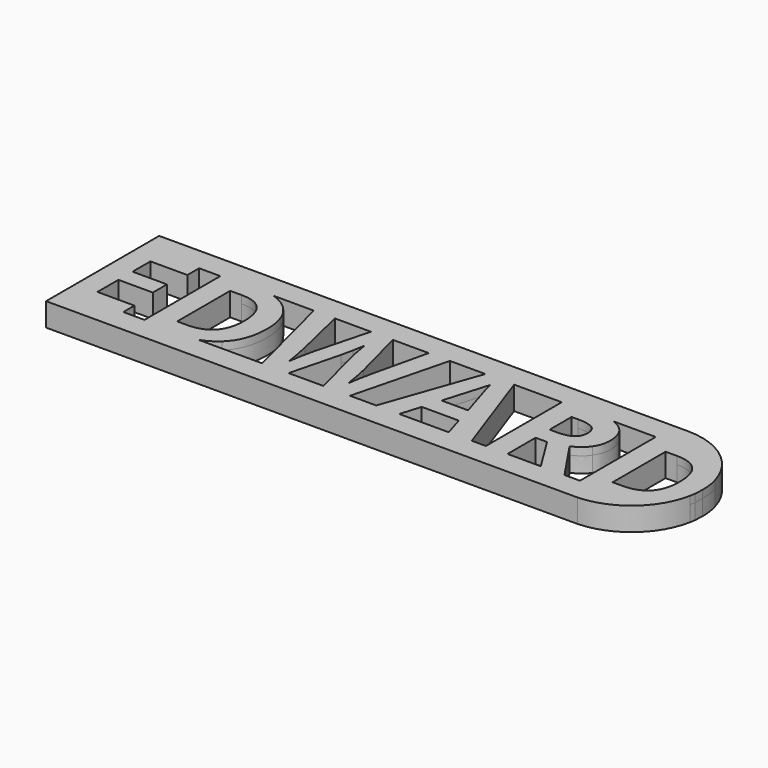
from build123d import *

# Parameters (mm, degrees)
F0_W     = 7.5354432192
F0_H     = 0.5
F0_W_2   = 2.7753114707
F0_H_2   = 0.3883001575
F1_DEPTH = 2
F2_DEPTH = 1.6468566519
F3_DEPTH = 1.6468566519
F5_DEPTH = 2
F6_DEPTH = 2
F7_DEPTH = 1


with BuildPart() as f1:
    # F0 (on Top) → F1 (new body)
    with BuildSketch(Plane.XY):
        with Locations((-34.5854217385, 0.25)):
            Rectangle(F0_W, F0_H)
        Polygon((-38.3531433481, 12.6977660032), (-38.3531433481, 0.5), (-30.8177001289, 0.5), (-30.8177001289, 2.29127882), (-35.5778318774, 2.29127882), (-35.5778318774, 5.6651868824), (-31.1470714593, 5.6651868824), (-31.1470714593, 7.9392811113), (-35.5778318774, 7.9392811113), (-35.5778318774, 10.8119719318), (-30.8177001289, 10.8119719318), (-30.8177001289, 12.6977660032), align=None)
        with BuildLine():
            Line((-38.3531433481, 0.5), (-40, 0.5))
            Line((-40, 0.5), (-40, -2.5))
            Line((-40, -2.5), (40, -2.5))
            Line((40, -2.5), (40, 0.5))
            Line((40, 0.5), (34.9300250632, 0.5))
            add(Edge.make_bspline(
                [(34.9300250632, 0.5), (33.5321767459, 0), (31.6597450952, 0)],
                knots=[0.460594463, 0.460594463, 0.460594463, 1, 1, 1], degree=2))
            Line((31.6597450952, 0), (27.9536016039, 0))
            Line((27.9536016039, 0), (27.9536016039, 0.5))
            Line((27.9536016039, 0.5), (25.9628201622, 0.5))
            add(Edge.make_bspline(
                [(25.9628201622, 0.5), (26.1618801681, 0.2089395921), (26.306744952, 0)],
                knots=[0.837886092, 0.837886092, 0.837886092, 1, 1, 1], degree=2))
            Line((26.306744952, 0), (23.2278390377, 0))
            Line((23.2278390377, 0), (22.9166582048, 0.5))
            Line((22.9166582048, 0.5), (18.6280968065, 0.5))
            Line((18.6280968065, 0.5), (18.6280968065, 0))
            Line((18.6280968065, 0), (15.8527853358, 0))
            Line((15.8527853358, 0), (15.8527853358, 0.5))
            Line((15.8527853358, 0.5), (14.0294901486, 0.5))
            Line((14.0294901486, 0.5), (14.2059286839, 0))
            Line((14.2059286839, 0), (11.2158098239, 0))
            Line((11.2158098239, 0), (11.0636958533, 0.5))
            Line((11.0636958533, 0.5), (4.7003024283, 0.5))
            Line((4.7003024283, 0.5), (4.5481884577, 0))
            Line((4.5481884577, 0), (1.5580695976, 0))
            Line((1.5580695976, 0), (1.7338542532, 0.5))
            Line((1.7338542532, 0.5), (-1.6456062494, 0.5))
            Line((-1.6456062494, 0.5), (-1.772876987, 0))
            Line((-1.772876987, 0), (-4.93197766, 0))
            Line((-4.93197766, 0), (-5.0609359934, 0.5))
            Line((-5.0609359934, 0.5), (-9.5464787021, 0.5))
            Line((-9.5464787021, 0.5), (-9.6749248174, 0))
            Line((-9.6749248174, 0), (-12.8254331949, 0))
            Line((-12.8254331949, 0), (-12.9530322319, 0.5))
            Line((-12.9530322319, 0.5), (-21.1117907752, 0.5))
            add(Edge.make_bspline(
                [(-21.1117907752, 0.5), (-22.5096390926, 0), (-24.3820707432, 0)],
                knots=[0.460594463, 0.460594463, 0.460594463, 1, 1, 1], degree=2))
            Line((-24.3820707432, 0), (-28.0882142346, 0))
            Line((-28.0882142346, 0), (-28.0882142346, 0.5))
            Line((-28.0882142346, 0.5), (-30.8177001289, 0.5))
            Line((-30.8177001289, 0.5), (-30.8177001289, 0))
            Line((-30.8177001289, 0), (-38.3531433481, 0))
            Line((-38.3531433481, 0), (-38.3531433481, 0.5))
        make_face()
        with BuildLine():
            Line((-28.0882142346, 12.6977660032), (-28.0882142346, 0.5))
            Line((-28.0882142346, 0.5), (-21.1117907752, 0.5))
            add(Edge.make_bspline(
                [(-19.0706000286, 1.718459115), (-19.9181782686, 0.9269463617), (-21.1117907752, 0.5)],
                knots=[0, 0, 0, 0.460594463, 0.460594463, 0.460594463], degree=2))
            add(Edge.make_bspline(
                [(-17.2304167263, 6.6676213662), (-17.2304167263, 3.43691823), (-19.0706000286, 1.718459115)],
                knots=[0, 0, 0, 1, 1, 1], degree=2))
            add(Edge.make_bspline(
                [(-19.0032937133, 11.3948159817), (-17.2304167263, 9.7035658027), (-17.2304167263, 6.6676213662)],
                knots=[0, 0, 0, 1, 1, 1], degree=2))
            add(Edge.make_bspline(
                [(-21.2385462766, 12.6977660032), (-19.9266803337, 12.2756880323), (-19.0032937133, 11.3948159817)],
                knots=[0.479159227, 0.479159227, 0.479159227, 1, 1, 1], degree=2))
            Line((-21.2385462766, 12.6977660032), (-28.0882142346, 12.6977660032))
        make_face()
        with BuildLine():
            add(Edge.make_bspline(
                [(-20.114563941, 6.5960189031), (-20.114563941, 10.8119719318), (-23.8378920235, 10.8119719318)],
                knots=[0, 0, 0, 1, 1, 1], degree=2))
            add(Edge.make_bspline(
                [(-24.124301876, 2.29127882), (-20.114563941, 2.29127882), (-20.114563941, 6.5960189031)],
                knots=[0, 0, 0, 1, 1, 1], degree=2))
            Line((-24.124301876, 2.29127882), (-25.3129027639, 2.29127882))
            Line((-25.3129027639, 2.29127882), (-25.3129027639, 10.8119719318))
            Line((-25.3129027639, 10.8119719318), (-23.8378920235, 10.8119719318))
        make_face(mode=Mode.SUBTRACT)
        with BuildLine():
            Line((-21.1117907752, 0.5), (-28.0882142346, 0.5))
            Line((-28.0882142346, 0.5), (-28.0882142346, 0))
            Line((-28.0882142346, 0), (-24.3820707432, 0))
            add(Edge.make_bspline(
                [(-21.1117907752, 0.5), (-22.5096390926, 0), (-24.3820707432, 0)],
                knots=[0.460594463, 0.460594463, 0.460594463, 1, 1, 1], degree=2))
        make_face()
        with BuildLine():
            Line((-16.0658786227, 12.6977660032), (-12.9530322319, 0.5))
            Line((-12.9530322319, 0.5), (-9.5464787021, 0.5))
            Line((-9.5464787021, 0.5), (-7.9135042245, 6.8566518688))
            add(Edge.make_bspline(
                [(-7.5812687956, 8.3817843334), (-7.796076185, 7.3120435343), (-7.9135042245, 6.8566518688)],
                knots=[0, 0, 0, 1, 1, 1], degree=2))
            add(Edge.make_bspline(
                [(-7.3120435343, 9.9355577832), (-7.3664614063, 9.4515251325), (-7.5812687956, 8.3817843334)],
                knots=[0, 0, 0, 1, 1, 1], degree=2))
            add(Edge.make_bspline(
                [(-7.0399541744, 8.390376629), (-7.277674352, 9.5403121867), (-7.3120435343, 9.9355577832)],
                knots=[0, 0, 0, 1, 1, 1], degree=2))
            add(Edge.make_bspline(
                [(-6.704854647, 6.87383646), (-6.8022339968, 7.2404410712), (-7.0399541744, 8.390376629)],
                knots=[0, 0, 0, 1, 1, 1], degree=2))
            Line((-6.704854647, 6.87383646), (-5.0609359934, 0.5))
            Line((-5.0609359934, 0.5), (-1.6456062494, 0.5))
            Line((-1.6456062494, 0.5), (1.4592311027, 12.6977660032))
            Line((1.4592311027, 12.6977660032), (-1.2647384512, 12.6977660032))
            Line((-1.2647384512, 12.6977660032), (-2.8383216383, 5.9430044394))
            add(Edge.make_bspline(
                [(-3.1963339539, 4.2560504081), (-2.9987111557, 5.2985822712), (-2.8383216383, 5.9430044394)],
                knots=[0, 0, 0, 1, 1, 1], degree=2))
            add(Edge.make_bspline(
                [(-3.4827438064, 2.5146785049), (-3.3939567521, 3.213518545), (-3.1963339539, 4.2560504081)],
                knots=[0, 0, 0, 1, 1, 1], degree=2))
            add(Edge.make_bspline(
                [(-3.7677216096, 4.2517542603), (-3.5801231562, 3.2392954318), (-3.4827438064, 2.5146785049)],
                knots=[0, 0, 0, 1, 1, 1], degree=2))
            add(Edge.make_bspline(
                [(-4.0813403981, 5.7539739367), (-3.955320063, 5.2642130889), (-3.7677216096, 4.2517542603)],
                knots=[0, 0, 0, 1, 1, 1], degree=2))
            Line((-4.0813403981, 5.7539739367), (-5.8878113029, 12.6977660032))
            Line((-5.8878113029, 12.6977660032), (-8.710498879, 12.6977660032))
            Line((-8.710498879, 12.6977660032), (-10.5169697838, 5.7539739367))
            add(Edge.make_bspline(
                [(-10.8792782472, 4.0942288415), (-10.6859515967, 5.1639696406), (-10.5169697838, 5.7539739367)],
                knots=[0, 0, 0, 1, 1, 1], degree=2))
            add(Edge.make_bspline(
                [(-11.1270227696, 2.5146785049), (-11.0726048976, 3.0244880424), (-10.8792782472, 4.0942288415)],
                knots=[0, 0, 0, 1, 1, 1], degree=2))
            add(Edge.make_bspline(
                [(-11.7599885436, 5.9430044394), (-11.3217814693, 3.9639123586), (-11.1270227696, 2.5146785049)],
                knots=[0, 0, 0, 1, 1, 1], degree=2))
            Line((-11.7599885436, 5.9430044394), (-13.3444053499, 12.6977660032))
            Line((-13.3444053499, 12.6977660032), (-16.0658786227, 12.6977660032))
        make_face()
        Polygon((-9.5464787021, 0.5), (-12.9530322319, 0.5), (-12.8254331949, 0), (-9.6749248174, 0), align=None)
        Polygon((-1.6456062494, 0.5), (-5.0609359934, 0.5), (-4.93197766, 0), (-1.772876987, 0), align=None)
        Polygon((6.0222144457, 12.6977660032), (1.7338542532, 0.5), (4.7003024283, 0.5), (5.4962050695, 3.1161391952), (10.2677932121, 3.1161391952), (11.0636958533, 0.5), (14.0294901486, 0.5), (9.7251782133, 12.6977660032), align=None)
        with BuildLine():
            add(Edge.make_bspline(
                [(9.6033223543, 5.4417871975), (8.2887011313, 9.6749248174), (8.1225834169, 10.2305599313)],
                knots=[0, 0, 0, 1, 1, 1], degree=2))
            Line((9.6033223543, 5.4417871975), (6.1950451096, 5.4417871975))
            add(Edge.make_bspline(
                [(7.8848632393, 11.1069740799), (7.5898610912, 9.9613346699), (6.1950451096, 5.4417871975)],
                knots=[0, 0, 0, 1, 1, 1], degree=2))
            add(Edge.make_bspline(
                [(8.1225834169, 10.2305599313), (7.9564657024, 10.7861950451), (7.8848632393, 11.1069740799)],
                knots=[0, 0, 0, 1, 1, 1], degree=2))
        make_face(mode=Mode.SUBTRACT)
        Polygon((4.7003024283, 0.5), (1.7338542532, 0.5), (1.5580695976, 0), (4.5481884577, 0), align=None)
        Polygon((14.2059286839, 0), (14.0294901486, 0.5), (11.0636958533, 0.5), (11.2158098239, 0), align=None)
        with BuildLine():
            Line((22.9166582048, 0.5), (25.9628201622, 0.5))
            add(Edge.make_bspline(
                [(22.4573965344, 5.7024201633), (24.9339780809, 2.0043463618), (25.9628201622, 0.5)],
                knots=[0, 0, 0, 0.837886092, 0.837886092, 0.837886092], degree=2))
            add(Edge.make_bspline(
                [(24.2574824574, 7.1115566375), (23.6230846341, 6.2122297007), (22.4573965344, 5.7024201633)],
                knots=[0, 0, 0, 1, 1, 1], degree=2))
            add(Edge.make_bspline(
                [(24.8918802807, 9.16511528), (24.8918802807, 8.0108835744), (24.2574824574, 7.1115566375)],
                knots=[0, 0, 0, 1, 1, 1], degree=2))
            add(Edge.make_bspline(
                [(23.6130602893, 12.1151367607), (24.8918802807, 11.1442073607), (24.8918802807, 9.16511528)],
                knots=[0, 0, 0, 1, 1, 1], degree=2))
            add(Edge.make_bspline(
                [(22.4849612957, 12.6977660032), (23.1429625152, 12.4720530998), (23.6130602893, 12.1151367607)],
                knots=[0.6323972278, 0.6323972278, 0.6323972278, 1, 1, 1], degree=2))
            Line((22.4849612957, 12.6977660032), (15.8527853358, 12.6977660032))
            Line((15.8527853358, 12.6977660032), (15.8527853358, 0.5))
            Line((15.8527853358, 0.5), (18.6280968065, 0.5))
            Line((18.6280968065, 0.5), (18.6280968065, 5.0207647143))
            Line((18.6280968065, 5.0207647143), (20.1031075469, 5.0207647143))
            Line((20.1031075469, 5.0207647143), (22.9166582048, 0.5))
        make_face()
        with BuildLine():
            Line((19.5216955463, 7.277674352), (18.6280968065, 7.277674352))
            Line((18.6280968065, 7.277674352), (18.6280968065, 10.8119719318))
            Line((18.6280968065, 10.8119719318), (19.4701417729, 10.8119719318))
            add(Edge.make_bspline(
                [(21.4506659029, 10.4181583846), (20.8105398826, 10.8119719318), (19.4701417729, 10.8119719318)],
                knots=[0, 0, 0, 1, 1, 1], degree=2))
            add(Edge.make_bspline(
                [(22.0907919232, 9.0935128168), (22.0907919232, 10.0243448375), (21.4506659029, 10.4181583846)],
                knots=[0, 0, 0, 1, 1, 1], degree=2))
            add(Edge.make_bspline(
                [(21.4649863955, 7.7158814263), (22.0907919232, 8.1540885006), (22.0907919232, 9.0935128168)],
                knots=[0, 0, 0, 1, 1, 1], degree=2))
            add(Edge.make_bspline(
                [(19.5216955463, 7.277674352), (20.8391808678, 7.277674352), (21.4649863955, 7.7158814263)],
                knots=[0, 0, 0, 1, 1, 1], degree=2))
        make_face(mode=Mode.SUBTRACT)
        with Locations((17.2404410712, 0.25)):
            Rectangle(F0_W_2, F0_H)
        with BuildLine():
            add(Edge.make_bspline(
                [(25.9628201622, 0.5), (26.1618801681, 0.2089395921), (26.306744952, 0)],
                knots=[0.837886092, 0.837886092, 0.837886092, 1, 1, 1], degree=2))
            Line((25.9628201622, 0.5), (22.9166582048, 0.5))
            Line((22.9166582048, 0.5), (23.2278390377, 0))
            Line((23.2278390377, 0), (26.306744952, 0))
        make_face()
        with BuildLine():
            add(Edge.make_bspline(
                [(34.9300250632, 0.5), (33.5321767459, 0), (31.6597450952, 0)],
                knots=[0.460594463, 0.460594463, 0.460594463, 1, 1, 1], degree=2))
            Line((34.9300250632, 0.5), (27.9536016039, 0.5))
            Line((27.9536016039, 0.5), (27.9536016039, 0))
            Line((27.9536016039, 0), (31.6597450952, 0))
        make_face()
        with BuildLine():
            Line((27.9536016039, 0.5), (34.9300250632, 0.5))
            add(Edge.make_bspline(
                [(36.9712158098, 1.718459115), (36.1236375699, 0.9269463617), (34.9300250632, 0.5)],
                knots=[0, 0, 0, 0.460594463, 0.460594463, 0.460594463], degree=2))
            add(Edge.make_bspline(
                [(38.8113991121, 6.6676213662), (38.8113991121, 3.43691823), (36.9712158098, 1.718459115)],
                knots=[0, 0, 0, 1, 1, 1], degree=2))
            add(Edge.make_bspline(
                [(37.0385221252, 11.3948159817), (38.8113991121, 9.7035658027), (38.8113991121, 6.6676213662)],
                knots=[0, 0, 0, 1, 1, 1], degree=2))
            add(Edge.make_bspline(
                [(34.8032695619, 12.6977660032), (36.1151355048, 12.2756880323), (37.0385221252, 11.3948159817)],
                knots=[0.479159227, 0.479159227, 0.479159227, 1, 1, 1], degree=2))
            Line((34.8032695619, 12.6977660032), (27.9536016039, 12.6977660032))
            Line((27.9536016039, 12.6977660032), (27.9536016039, 0.5))
        make_face()
        with BuildLine():
            add(Edge.make_bspline(
                [(35.9272518975, 6.5960189031), (35.9272518975, 10.8119719318), (32.203923815, 10.8119719318)],
                knots=[0, 0, 0, 1, 1, 1], degree=2))
            add(Edge.make_bspline(
                [(31.9175139625, 2.29127882), (35.9272518975, 2.29127882), (35.9272518975, 6.5960189031)],
                knots=[0, 0, 0, 1, 1, 1], degree=2))
            Line((31.9175139625, 2.29127882), (30.7289130746, 2.29127882))
            Line((30.7289130746, 2.29127882), (30.7289130746, 10.8119719318))
            Line((30.7289130746, 10.8119719318), (32.203923815, 10.8119719318))
        make_face(mode=Mode.SUBTRACT)
        with BuildLine():
            Line((-40, 12.6977660032), (-38.3531433481, 12.6977660032))
            Line((-38.3531433481, 12.6977660032), (-38.3531433481, 13.0860661607))
            Line((-38.3531433481, 13.0860661607), (-30.8177001289, 13.0860661607))
            Line((-30.8177001289, 13.0860661607), (-30.8177001289, 12.6977660032))
            Line((-30.8177001289, 12.6977660032), (-28.0882142346, 12.6977660032))
            Line((-28.0882142346, 12.6977660032), (-28.0882142346, 13.0860661607))
            Line((-28.0882142346, 13.0860661607), (-23.9810969497, 13.0860661607))
            add(Edge.make_bspline(
                [(-23.9810969497, 13.0860661607), (-22.4454269656, 13.0860661607), (-21.2385462766, 12.6977660032)],
                knots=[0, 0, 0, 0.479159227, 0.479159227, 0.479159227], degree=2))
            Line((-21.2385462766, 12.6977660032), (-16.0658786227, 12.6977660032))
            Line((-16.0658786227, 12.6977660032), (-16.164972075, 13.0860661607))
            Line((-16.164972075, 13.0860661607), (-13.4354861807, 13.0860661607))
            Line((-13.4354861807, 13.0860661607), (-13.3444053499, 12.6977660032))
            Line((-13.3444053499, 12.6977660032), (-8.710498879, 12.6977660032))
            Line((-8.710498879, 12.6977660032), (-8.6094801661, 13.0860661607))
            Line((-8.6094801661, 13.0860661607), (-5.9888300158, 13.0860661607))
            Line((-5.9888300158, 13.0860661607), (-5.8878113029, 12.6977660032))
            Line((-5.8878113029, 12.6977660032), (-1.2647384512, 12.6977660032))
            Line((-1.2647384512, 12.6977660032), (-1.1742803952, 13.0860661607))
            Line((-1.1742803952, 13.0860661607), (1.5580695976, 13.0860661607))
            Line((1.5580695976, 13.0860661607), (1.4592311027, 12.6977660032))
            Line((1.4592311027, 12.6977660032), (6.0222144457, 12.6977660032))
            Line((6.0222144457, 12.6977660032), (6.1778605184, 13.1404840327))
            Line((6.1778605184, 13.1404840327), (9.568953172, 13.1404840327))
            Line((9.568953172, 13.1404840327), (9.7251782133, 12.6977660032))
            Line((9.7251782133, 12.6977660032), (15.8527853358, 12.6977660032))
            Line((15.8527853358, 12.6977660032), (15.8527853358, 13.0860661607))
            Line((15.8527853358, 13.0860661607), (19.6649004726, 13.0860661607))
            add(Edge.make_bspline(
                [(19.6649004726, 13.0860661607), (21.3529835781, 13.0860661607), (22.4849612957, 12.6977660032)],
                knots=[0, 0, 0, 0.6323972278, 0.6323972278, 0.6323972278], degree=2))
            Line((22.4849612957, 12.6977660032), (27.9536016039, 12.6977660032))
            Line((27.9536016039, 12.6977660032), (27.9536016039, 13.0860661607))
            Line((27.9536016039, 13.0860661607), (32.0607188887, 13.0860661607))
            add(Edge.make_bspline(
                [(32.0607188887, 13.0860661607), (33.5963888729, 13.0860661607), (34.8032695619, 12.6977660032)],
                knots=[0, 0, 0, 0.479159227, 0.479159227, 0.479159227], degree=2))
            Line((34.8032695619, 12.6977660032), (40, 12.6977660032))
            Line((40, 12.6977660032), (40, 15.6977660032))
            Line((40, 15.6977660032), (-40, 15.6977660032))
            Line((-40, 15.6977660032), (-40, 12.6977660032))
        make_face()
        with BuildLine():
            Line((27.9536016039, 13.0860661607), (27.9536016039, 12.6977660032))
            Line((27.9536016039, 12.6977660032), (34.8032695619, 12.6977660032))
            add(Edge.make_bspline(
                [(32.0607188887, 13.0860661607), (33.5963888729, 13.0860661607), (34.8032695619, 12.6977660032)],
                knots=[0, 0, 0, 0.479159227, 0.479159227, 0.479159227], degree=2))
            Line((32.0607188887, 13.0860661607), (27.9536016039, 13.0860661607))
        make_face()
        with BuildLine():
            Line((15.8527853358, 12.6977660032), (22.4849612957, 12.6977660032))
            add(Edge.make_bspline(
                [(19.6649004726, 13.0860661607), (21.3529835781, 13.0860661607), (22.4849612957, 12.6977660032)],
                knots=[0, 0, 0, 0.6323972278, 0.6323972278, 0.6323972278], degree=2))
            Line((19.6649004726, 13.0860661607), (15.8527853358, 13.0860661607))
            Line((15.8527853358, 13.0860661607), (15.8527853358, 12.6977660032))
        make_face()
        Polygon((6.0222144457, 12.6977660032), (9.7251782133, 12.6977660032), (9.568953172, 13.1404840327), (6.1778605184, 13.1404840327), align=None)
        Polygon((-1.2647384512, 12.6977660032), (1.4592311027, 12.6977660032), (1.5580695976, 13.0860661607), (-1.1742803952, 13.0860661607), align=None)
        Polygon((-8.6094801661, 13.0860661607), (-8.710498879, 12.6977660032), (-5.8878113029, 12.6977660032), (-5.9888300158, 13.0860661607), align=None)
        Polygon((-16.164972075, 13.0860661607), (-16.0658786227, 12.6977660032), (-13.3444053499, 12.6977660032), (-13.4354861807, 13.0860661607), align=None)
        with BuildLine():
            Line((-28.0882142346, 13.0860661607), (-28.0882142346, 12.6977660032))
            Line((-28.0882142346, 12.6977660032), (-21.2385462766, 12.6977660032))
            add(Edge.make_bspline(
                [(-23.9810969497, 13.0860661607), (-22.4454269656, 13.0860661607), (-21.2385462766, 12.6977660032)],
                knots=[0, 0, 0, 0.479159227, 0.479159227, 0.479159227], degree=2))
            Line((-23.9810969497, 13.0860661607), (-28.0882142346, 13.0860661607))
        make_face()
        with Locations((-34.5854217385, 12.8919160819)):
            Rectangle(F0_W, F0_H_2)
    extrude(amount=F1_DEPTH)

    # F2 (cut, through all): a face of the model
    f2_faces = [f1.faces().sort_by_distance(p)[0] for p in [
        (-40, 14.1977660032, 1),
    ]]
    extrude(f2_faces, amount=-F2_DEPTH, mode=Mode.SUBTRACT)

    # F3 (cut, through all): a face of the model
    f3_faces = [f1.faces().sort_by_distance(p)[0] for p in [
        (-40, -1, 1),
    ]]
    extrude(f3_faces, amount=-F3_DEPTH, mode=Mode.SUBTRACT)

    # F4 (on face) → F5 (join, through all)
    with BuildSketch(Plane.XY.offset(2)):
        with BuildLine():
            add(Edge.make_bspline(
                [(38.7514867962, 5.5509748014), (38.8113991121, 6.0846804162), (38.8113991121, 6.6676213662)],
                knots=[1.2801566681, 1.2801566681, 1.2801566681, 1.460594463, 1.460594463, 1.460594463], degree=2))
            ThreePointArc((38.8113991121, 6.6676213662), (38.7165601523, 7.9084515742), (38.4533502929, 9.1247470166))
            add(Edge.make_bspline(
                [(38.4533502929, 9.1247470166), (38.0146704809, 10.4636114517), (36.1151355048, 12.2756880323), (34.8032695619, 12.6977660032)],
                knots=[1.8829017616, 1.8829017616, 1.8829017616, 2.4003107751, 2.8897533455, 2.8897533455, 2.8897533455], degree=2))
            Line((34.8032695619, 12.6977660032), (36.4634869923, 12.6977660032))
            ThreePointArc((36.4634869923, 12.6977660032), (33.4048789446, 14.9140222466), (29.7099336608, 15.6977660032))
            ThreePointArc((29.7099336608, 15.6977660032), (26.014988377, 14.9140222466), (22.9563803294, 12.6977660032))
            Line((22.9563803294, 12.6977660032), (27.9536016039, 12.6977660032))
            Line((27.9536016039, 12.6977660032), (27.9536016039, 0.5))
            Line((27.9536016039, 0.5), (25.9628201622, 0.5))
            add(Edge.make_bspline(
                [(22.4573965344, 5.7024201633), (24.9339780809, 2.0043463618), (25.9628201622, 0.5)],
                knots=[0, 0, 0, 0.837886092, 0.837886092, 0.837886092], degree=2))
            add(Edge.make_bspline(
                [(22.4573965344, 5.7024201633), (23.6230846341, 6.2122297007), (24.8918802807, 8.0108835744), (24.8918802807, 11.1442073607), (23.2736431691, 12.3728353133), (22.8362712218, 12.5621369834)],
                knots=[0, 0, 0, 1, 2, 3.7146401985, 4.1697302363, 4.1697302363, 4.1697302363], degree=2))
            ThreePointArc((22.8362712218, 12.5621369834), (22.0675343598, 11.5392499514), (21.4498390087, 10.4186667566))
            add(Edge.make_bspline(
                [(21.4498390087, 10.4186667566), (21.4502526018, 10.4184126527), (22.0907919232, 10.0243448375), (22.0907919232, 8.1540885006), (21.1443616579, 7.4913707405), (20.6421768454, 7.3818856921)],
                knots=[0.9993543441, 0.9993543441, 0.9993543441, 1, 2, 3.0092307692, 3.5262993094, 3.5262993094, 3.5262993094], degree=2))
            ThreePointArc((20.6421768454, 7.3818856921), (20.7189867364, 5.1801539105), (21.322556837, 3.0613746083))
            Line((21.322556837, 3.0613746083), (22.8346504374, 0.6317686675))
            ThreePointArc((22.8346504374, 0.6317686675), (25.7849724762, -1.6159528439), (29.3870708579, -2.5))
            Line((29.3870708579, -2.5), (30.0327964638, -2.5))
            ThreePointArc((30.0327964638, -2.5), (33.5553489675, -1.6535011674), (36.4686579345, 0.5))
            Line((36.4686579345, 0.5), (34.9300250632, 0.5))
            add(Edge.make_bspline(
                [(34.9300250632, 0.5), (36.1236375699, 0.9269463617), (38.2492112013, 2.9119178463), (38.6396470662, 4.8347640174)],
                knots=[0, 0, 0, 0.460594463, 1.1550879898, 1.1550879898, 1.1550879898], degree=2))
            ThreePointArc((38.6396470662, 4.8347640174), (38.702699906, 5.1917555614), (38.7514867962, 5.5509748014))
        make_face()
        with BuildLine():
            add(Edge.make_bspline(
                [(32.203923815, 10.8119719318), (35.9272518975, 10.8119719318), (35.9272518975, 2.29127882), (31.9175139625, 2.29127882)],
                knots=[0, 0, 0, 1, 2.0210597826, 2.0210597826, 2.0210597826], degree=2))
            Line((31.9175139625, 2.29127882), (30.7289130746, 2.29127882))
            Line((30.7289130746, 2.29127882), (30.7289130746, 10.8119719318))
            Line((30.7289130746, 10.8119719318), (32.203923815, 10.8119719318))
        make_face(mode=Mode.SUBTRACT)
        with BuildLine():
            add(Edge.make_bspline(
                [(38.4533502929, 9.1247470166), (38.0146704809, 10.4636114517), (36.1151355048, 12.2756880323), (34.8032695619, 12.6977660032)],
                knots=[1.8829017616, 1.8829017616, 1.8829017616, 2.4003107751, 2.8897533455, 2.8897533455, 2.8897533455], degree=2))
            ThreePointArc((38.4533502929, 9.1247470166), (37.6617030037, 11.0244683599), (36.4634869923, 12.6977660032))
            Line((36.4634869923, 12.6977660032), (34.8032695619, 12.6977660032))
        make_face()
        with BuildLine():
            ThreePointArc((36.4686579345, 0.5), (37.8480731272, 2.5201771127), (38.6396470662, 4.8347640174))
            add(Edge.make_bspline(
                [(34.9300250632, 0.5), (36.1236375699, 0.9269463617), (38.2492112013, 2.9119178463), (38.6396470662, 4.8347640174)],
                knots=[0, 0, 0, 0.460594463, 1.1550879898, 1.1550879898, 1.1550879898], degree=2))
            Line((34.9300250632, 0.5), (36.4686579345, 0.5))
        make_face()
    extrude(amount=-F5_DEPTH)

    # F4 (on face) → F6 (cut, through all)
    with BuildSketch(Plane.XY.offset(2)):
        with BuildLine():
            ThreePointArc((29.7099336608, 15.6977660032), (33.4048789446, 14.9140222466), (36.4634869923, 12.6977660032))
            Line((36.4634869923, 12.6977660032), (40, 12.6977660032))
            Line((40, 12.6977660032), (40, 15.6977660032))
            Line((40, 15.6977660032), (29.7099336608, 15.6977660032))
        make_face()
        with BuildLine():
            Line((40, 0.5), (36.4686579345, 0.5))
            ThreePointArc((36.4686579345, 0.5), (33.5553489675, -1.6535011674), (30.0327964638, -2.5))
            Line((30.0327964638, -2.5), (40, -2.5))
            Line((40, -2.5), (40, 0.5))
        make_face()
    extrude(amount=-F6_DEPTH, mode=Mode.SUBTRACT)

    # F7 (add): a face of the model
    f7_faces = [f1.faces().sort_by_distance(p)[0] for p in [
        (-0.8641700918, 6.5908455777, 2),
    ]]
    extrude(f7_faces, amount=F7_DEPTH)


solid = f1.part
